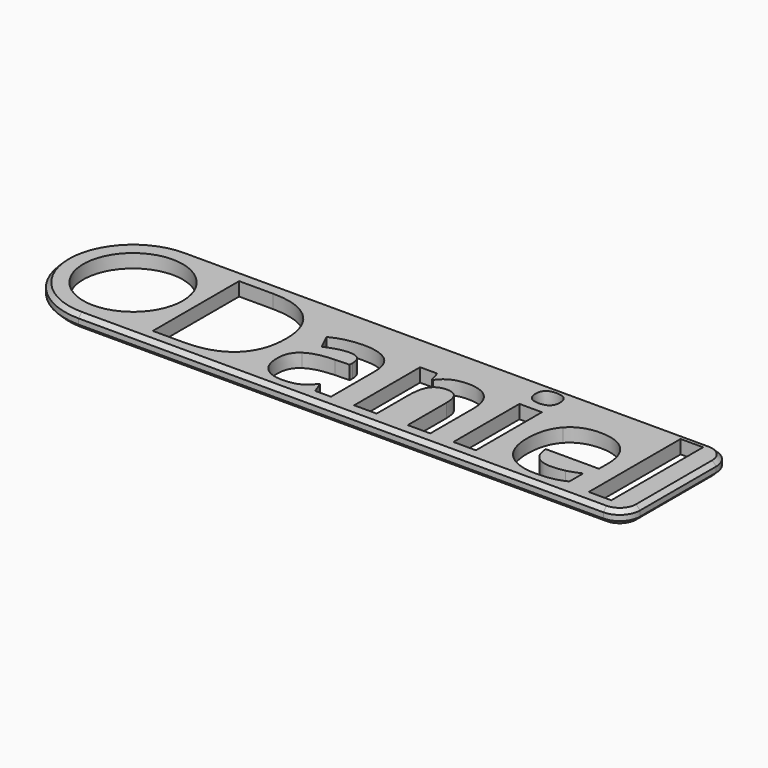
from build123d import *

# Parameters (mm, degrees)
F0_W     = 3.3090277778
F0_H     = 12.1319444444
F0_R     = 7.3151249886
F0_H_2   = 16.8854166667
F1_DEPTH = 2
F2_SIZE  = 0.6


with BuildPart() as f1:
    # F0 (on Top) → F1 (new body)
    with BuildSketch(Plane.XY):
        with BuildLine():
            Line((40.2255926098, 10), (-36.9645323787, 10))
            ThreePointArc((-36.9645323787, 10), (-46.9645323787, 0), (-36.9645323787, -10))
            Line((-36.9645323787, -10), (40.2255926098, -10))
            ThreePointArc((40.2255926098, -10), (42.3469129534, -9.1213203436), (43.2255926098, -7))
            Line((43.2255926098, -7), (43.2255926098, 7))
            ThreePointArc((43.2255926098, 7), (42.3469129534, 9.1213203436), (40.2255926098, 10))
        make_face()
        with BuildLine():
            add(Edge.make_bspline(
                [(-16.6389907235, 5.8142361111), (-14.4896851679, 3.7638888889), (-14.4896851679, 0.0833333333)],
                knots=[0, 0, 0, 1, 1, 1], degree=2))
            add(Edge.make_bspline(
                [(-14.4896851679, 0.0833333333), (-14.4896851679, -3.8333333333), (-16.7205879457, -5.9166666667)],
                knots=[0, 0, 0, 1, 1, 1], degree=2))
            add(Edge.make_bspline(
                [(-16.7205879457, -5.9166666667), (-18.9514907235, -8), (-23.1598240568, -8)],
                knots=[0, 0, 0, 1, 1, 1], degree=2))
            Line((-23.1598240568, -8), (-27.6528796124, -8))
            Line((-27.6528796124, -8), (-27.6528796124, 7.8645833333))
            Line((-27.6528796124, 7.8645833333), (-22.6737129457, 7.8645833333))
            add(Edge.make_bspline(
                [(-22.6737129457, 7.8645833333), (-18.7882962791, 7.8645833333), (-16.6389907235, 5.8142361111)],
                knots=[0, 0, 0, 1, 1, 1], degree=2))
        make_face(mode=Mode.SUBTRACT)
        with BuildLine():
            Line((-1.4480185013, -8), (-3.7570462791, -8))
            Line((-3.7570462791, -8), (-4.3994073902, -6.3506944444))
            Line((-4.3994073902, -6.3506944444), (-4.4862129457, -6.3506944444))
            add(Edge.make_bspline(
                [(-4.4862129457, -6.3506944444), (-5.3195462791, -7.4027777778), (-6.2049629457, -7.8107638889)],
                knots=[0, 0, 0, 1, 1, 1], degree=2))
            add(Edge.make_bspline(
                [(-6.2049629457, -7.8107638889), (-7.0903796124, -8.21875), (-8.5105185013, -8.21875)],
                knots=[0, 0, 0, 1, 1, 1], degree=2))
            add(Edge.make_bspline(
                [(-8.5105185013, -8.21875), (-10.2570462791, -8.21875), (-11.2605185013, -7.21875)],
                knots=[0, 0, 0, 1, 1, 1], degree=2))
            add(Edge.make_bspline(
                [(-11.2605185013, -7.21875), (-12.2639907235, -6.21875), (-12.2639907235, -4.375)],
                knots=[0, 0, 0, 1, 1, 1], degree=2))
            add(Edge.make_bspline(
                [(-12.2639907235, -4.375), (-12.2639907235, -2.4444444444), (-10.9132962791, -1.5277777778)],
                knots=[0, 0, 0, 1, 1, 1], degree=2))
            add(Edge.make_bspline(
                [(-10.9132962791, -1.5277777778), (-9.5626018346, -0.6111111111), (-6.8403796124, -0.5138888889)],
                knots=[0, 0, 0, 1, 1, 1], degree=2))
            Line((-6.8403796124, -0.5138888889), (-4.7327407235, -0.4479166667))
            Line((-4.7327407235, -0.4479166667), (-4.7327407235, 0.0833333333))
            add(Edge.make_bspline(
                [(-4.7327407235, 0.0833333333), (-4.7327407235, 1.9270833333), (-6.6216296124, 1.9270833333)],
                knots=[0, 0, 0, 1, 1, 1], degree=2))
            add(Edge.make_bspline(
                [(-6.6216296124, 1.9270833333), (-8.0764907235, 1.9270833333), (-10.0417685013, 1.0486111111)],
                knots=[0, 0, 0, 1, 1, 1], degree=2))
            Line((-10.0417685013, 1.0486111111), (-11.1355185013, 3.2847222222))
            add(Edge.make_bspline(
                [(-11.1355185013, 3.2847222222), (-9.0417685013, 4.3819444444), (-6.4931573902, 4.3819444444)],
                knots=[0, 0, 0, 1, 1, 1], degree=2))
            add(Edge.make_bspline(
                [(-6.4931573902, 4.3819444444), (-4.0521851679, 4.3819444444), (-2.7501018346, 3.3177083333)],
                knots=[0, 0, 0, 1, 1, 1], degree=2))
            add(Edge.make_bspline(
                [(-2.7501018346, 3.3177083333), (-1.4480185013, 2.2534722222), (-1.4480185013, 0.0833333333)],
                knots=[0, 0, 0, 1, 1, 1], degree=2))
            Line((-1.4480185013, 0.0833333333), (-1.4480185013, -8))
        make_face(mode=Mode.SUBTRACT)
        with BuildLine():
            Line((13.1596203876, -0.0902777778), (13.1596203876, -8))
            Line((13.1596203876, -8), (9.8505926098, -8))
            Line((9.8505926098, -8), (9.8505926098, -0.9131944444))
            add(Edge.make_bspline(
                [(9.8505926098, -0.9131944444), (9.8505926098, 0.3993055556), (9.3835787209, 1.0555555556)],
                knots=[0, 0, 0, 1, 1, 1], degree=2))
            add(Edge.make_bspline(
                [(9.3835787209, 1.0555555556), (8.9165648321, 1.7118055556), (7.8957314987, 1.7118055556)],
                knots=[0, 0, 0, 1, 1, 1], degree=2))
            add(Edge.make_bspline(
                [(7.8957314987, 1.7118055556), (6.5068426098, 1.7118055556), (5.8887870543, 0.7847222222)],
                knots=[0, 0, 0, 1, 1, 1], degree=2))
            add(Edge.make_bspline(
                [(5.8887870543, 0.7847222222), (5.2707314987, -0.1423611111), (5.2707314987, -2.2916666667)],
                knots=[0, 0, 0, 1, 1, 1], degree=2))
            Line((5.2707314987, -2.2916666667), (5.2707314987, -8))
            Line((5.2707314987, -8), (1.9617037209, -8))
            Line((1.9617037209, -8), (1.9617037209, 4.1319444444))
            Line((1.9617037209, 4.1319444444), (4.4894814987, 4.1319444444))
            Line((4.4894814987, 4.1319444444), (4.9339259432, 2.5798611111))
            Line((4.9339259432, 2.5798611111), (5.1179537209, 2.5798611111))
            add(Edge.make_bspline(
                [(5.1179537209, 2.5798611111), (5.6735092765, 3.4583333333), (6.6439953876, 3.9079861111)],
                knots=[0, 0, 0, 1, 1, 1], degree=2))
            add(Edge.make_bspline(
                [(6.6439953876, 3.9079861111), (7.6144814987, 4.3576388889), (8.8505926098, 4.3576388889)],
                knots=[0, 0, 0, 1, 1, 1], degree=2))
            add(Edge.make_bspline(
                [(8.8505926098, 4.3576388889), (10.9686481654, 4.3576388889), (12.0641342765, 3.2135416667)],
                knots=[0, 0, 0, 1, 1, 1], degree=2))
            add(Edge.make_bspline(
                [(12.0641342765, 3.2135416667), (13.1596203876, 2.0694444444), (13.1596203876, -0.0902777778)],
                knots=[0, 0, 0, 1, 1, 1], degree=2))
        make_face(mode=Mode.SUBTRACT)
        with Locations((18.2203842765, -1.9340277778)):
            Rectangle(F0_W, F0_H, mode=Mode.SUBTRACT)
        with BuildLine():
            add(Edge.make_bspline(
                [(31.2464259432, -8.0069444444), (30.2603148321, -8.21875), (28.8367037209, -8.21875)],
                knots=[0, 0, 0, 1, 1, 1], degree=2))
            add(Edge.make_bspline(
                [(28.8367037209, -8.21875), (25.9096203876, -8.21875), (24.2603148321, -6.6006944444)],
                knots=[0, 0, 0, 1, 1, 1], degree=2))
            add(Edge.make_bspline(
                [(24.2603148321, -6.6006944444), (22.6110092765, -4.9826388889), (22.6110092765, -2.0208333333)],
                knots=[0, 0, 0, 1, 1, 1], degree=2))
            add(Edge.make_bspline(
                [(22.6110092765, -2.0208333333), (22.6110092765, 1.0277777778), (24.1353148321, 2.6927083333)],
                knots=[0, 0, 0, 1, 1, 1], degree=2))
            add(Edge.make_bspline(
                [(24.1353148321, 2.6927083333), (25.6596203876, 4.3576388889), (28.3505926098, 4.3576388889)],
                knots=[0, 0, 0, 1, 1, 1], degree=2))
            add(Edge.make_bspline(
                [(28.3505926098, 4.3576388889), (30.9200370543, 4.3576388889), (32.3523287209, 2.8940972222)],
                knots=[0, 0, 0, 1, 1, 1], degree=2))
            add(Edge.make_bspline(
                [(32.3523287209, 2.8940972222), (33.7846203876, 1.4305555556), (33.7846203876, -1.1527777778)],
                knots=[0, 0, 0, 1, 1, 1], degree=2))
            Line((33.7846203876, -1.1527777778), (33.7846203876, -2.7604166667))
            Line((33.7846203876, -2.7604166667), (25.9617037209, -2.7604166667))
            add(Edge.make_bspline(
                [(25.9617037209, -2.7604166667), (26.0172592765, -4.1701388889), (26.7985092765, -4.9618055556)],
                knots=[0, 0, 0, 1, 1, 1], degree=2))
            add(Edge.make_bspline(
                [(26.7985092765, -4.9618055556), (27.5797592765, -5.7534722222), (28.9894814987, -5.7534722222)],
                knots=[0, 0, 0, 1, 1, 1], degree=2))
            add(Edge.make_bspline(
                [(28.9894814987, -5.7534722222), (30.0867037209, -5.7534722222), (31.0623981654, -5.5260416667)],
                knots=[0, 0, 0, 1, 1, 1], degree=2))
            add(Edge.make_bspline(
                [(31.0623981654, -5.5260416667), (32.0380926098, -5.2986111111), (33.1005926098, -4.7986111111)],
                knots=[0, 0, 0, 1, 1, 1], degree=2))
            Line((33.1005926098, -4.7986111111), (33.1005926098, -7.3611111111))
            add(Edge.make_bspline(
                [(33.1005926098, -7.3611111111), (32.2325370543, -7.7951388889), (31.2464259432, -8.0069444444)],
                knots=[0, 0, 0, 1, 1, 1], degree=2))
        make_face(mode=Mode.SUBTRACT)
        with Locations((-36.9645323787, 0)):
            Circle(F0_R, mode=Mode.SUBTRACT)
        with Locations((38.1301064987, 0.4427083333)):
            Rectangle(F0_W, F0_H_2, mode=Mode.SUBTRACT)
        with BuildLine():
            add(Edge.make_bspline(
                [(18.2255926098, 5.6388888889), (16.4235092765, 5.6388888889), (16.4235092765, 7.2673611111)],
                knots=[0, 0, 0, 1, 1, 1], degree=2))
            add(Edge.make_bspline(
                [(16.4235092765, 7.2673611111), (16.4235092765, 8.8854166667), (18.2255926098, 8.8854166667)],
                knots=[0, 0, 0, 1, 1, 1], degree=2))
            add(Edge.make_bspline(
                [(18.2255926098, 8.8854166667), (20.0276759432, 8.8854166667), (20.0276759432, 7.2673611111)],
                knots=[0, 0, 0, 1, 1, 1], degree=2))
            add(Edge.make_bspline(
                [(20.0276759432, 7.2673611111), (20.0276759432, 6.4965277778), (19.5780231654, 6.0677083333)],
                knots=[0, 0, 0, 1, 1, 1], degree=2))
            add(Edge.make_bspline(
                [(19.5780231654, 6.0677083333), (19.1283703876, 5.6388888889), (18.2255926098, 5.6388888889)],
                knots=[0, 0, 0, 1, 1, 1], degree=2))
        make_face(mode=Mode.SUBTRACT)
    extrude(amount=F1_DEPTH)

    # F2
    f2_edges = [f1.edges().sort_by_distance(p)[0] for p in [
        (1.63053, 10, 2),
        (1.63053, 10, 0),
    ]]
    chamfer(f2_edges, length=F2_SIZE)


solid = f1.part
